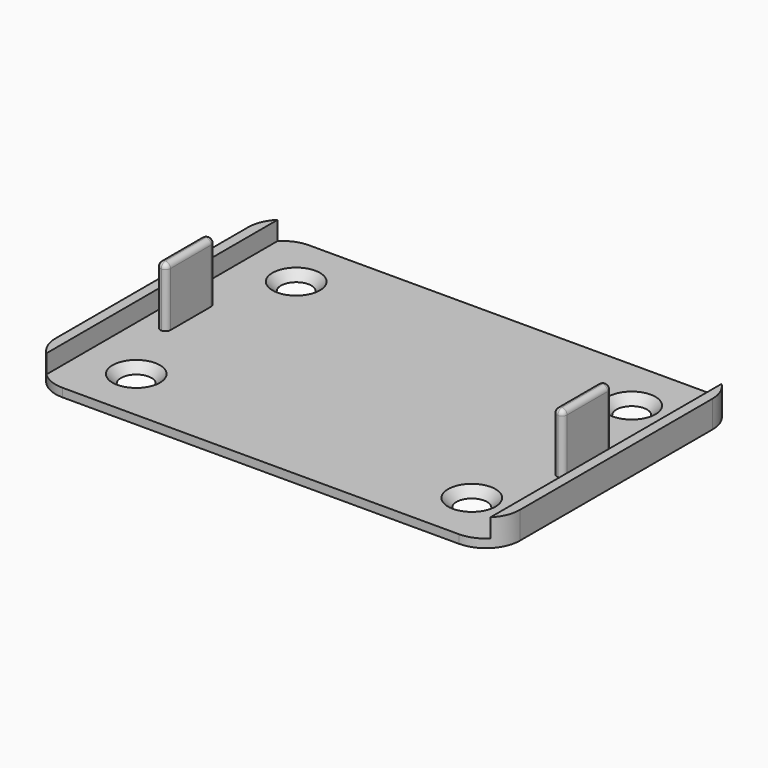
from build123d import *

# Parameters (mm, degrees)
F0_W     = 65.5
F0_H     = 45.5
F0_R     = 1.5
F0_W_2   = 1.5
F0_H_2   = 9
F1_DEPTH = 1.25
F2_DEPTH = 10
F3_DEPTH = 4
F5_R     = 0.74999
F6_R     = 0.74999
F7_R     = 5


# Not quite as in the source:
# - a fillet or chamfer that OpenCascade refuses, or shapes differently, is made with other operations: its cross-section is extruded or revolved along the edge and cut away or added
# - a fillet or chamfer is up to 0.001 mm smaller than in the source, because OpenCascade refuses the exact size


with BuildPart() as f1:
    # F0 (on Top) → F1 (new body)
    with BuildSketch(Plane.XY):
        Rectangle(F0_W, F0_H)
        with Locations((-24.75, -14.75)):
            Circle(F0_R, mode=Mode.SUBTRACT)
        with Locations((24.75, -14.75)):
            Circle(F0_R, mode=Mode.SUBTRACT)
        with Locations((-29.25, 0)):
            Rectangle(F0_W_2, F0_H_2, mode=Mode.SUBTRACT)
        with Locations((-24.75, 14.75)):
            Circle(F0_R, mode=Mode.SUBTRACT)
        with Locations((29.25, 0)):
            Rectangle(F0_W_2, F0_H_2, mode=Mode.SUBTRACT)
        with Locations((24.75, 14.75)):
            Circle(F0_R, mode=Mode.SUBTRACT)
    extrude(amount=F1_DEPTH)

    # F0 (on Top) → F2 (join)
    with BuildSketch(Plane.XY):
        with Locations((-29.25, 0)):
            Rectangle(F0_W_2, F0_H_2)
        with Locations((29.25, 0)):
            Rectangle(F0_W_2, F0_H_2)
    extrude(amount=F2_DEPTH)

    # F0 (on Top) → F3 (join)
    with BuildSketch(Plane.XY):
        with Locations((-33.5, 0)):
            Rectangle(F0_W_2, F0_H)
        with Locations((33.5, 0)):
            Rectangle(F0_W_2, F0_H)
    extrude(amount=F3_DEPTH)

    # F4: chamfer of 2 on 4 edges, made by hand

    # F4_s1 → F4_t2 (revolve, cut)
    with BuildSketch(Plane.XZ.offset(-14.75)):
        Polygon((-21.25, 1.25), (-23.25, -0.75), (-23.25, 1.25), align=None)
    revolve(axis=Axis((-24.75, 14.75, 1.25), (0, 0, 1)), mode=Mode.SUBTRACT)

    # F4_s3 → F4_t4 (revolve, cut)
    with BuildSketch(Plane.XZ.offset(14.75)):
        Polygon((-21.25, 1.25), (-23.25, -0.75), (-23.25, 1.25), align=None)
    revolve(axis=Axis((-24.75, -14.75, 1.25), (0, 0, 1)), mode=Mode.SUBTRACT)

    # F4_s5 → F4_t6 (revolve, cut)
    with BuildSketch(Plane.XZ.offset(-14.75)):
        Polygon((28.25, 1.25), (26.25, -0.75), (26.25, 1.25), align=None)
    revolve(axis=Axis((24.75, 14.75, 1.25), (0, 0, 1)), mode=Mode.SUBTRACT)

    # F4_s7 → F4_t8 (revolve, cut)
    with BuildSketch(Plane.XZ.offset(14.75)):
        Polygon((28.25, 1.25), (26.25, -0.75), (26.25, 1.25), align=None)
    revolve(axis=Axis((24.75, -14.75, 1.25), (0, 0, 1)), mode=Mode.SUBTRACT)

    # F5 (radius 0.75 in the source; OpenCascade refuses exactly that, so slightly less here)
    f5_edges = [f1.edges().sort_by_distance(p)[0] for p in [
        (-30, 4.5, 5.625),
        (30, 4.5, 5.625),
        (28.5, 4.5, 5.625),
        (-30, -4.5, 5.625),
        (-28.5, -4.5, 5.625),
        (28.5, -4.5, 5.625),
        (30, -4.5, 5.625),
        (-28.5, 4.5, 5.625),
    ]]
    fillet(f5_edges, radius=F5_R)

    # F6 (radius 0.75 in the source; OpenCascade refuses exactly that, so slightly less here)
    f6_edges = [f1.edges().sort_by_distance(p)[0] for p in [
        (-29.25, -4.5, 10),
        (-29.780333, -4.280333, 10),
        (-28.719667, -4.280333, 10),
        (-30, 0, 10),
        (-28.5, 0, 10),
        (-29.780333, 4.280333, 10),
        (-28.719667, 4.280333, 10),
        (-29.25, 4.5, 10),
        (29.25, -4.5, 10),
        (28.719667, -4.280333, 10),
        (29.780333, -4.280333, 10),
        (28.5, 0, 10),
        (30, 0, 10),
        (28.719667, 4.280333, 10),
        (29.780333, 4.280333, 10),
        (29.25, 4.5, 10),
    ]]
    fillet(f6_edges, radius=F6_R)

    # F7
    f7_edges = [f1.edges().sort_by_distance(p)[0] for p in [
        (-34.25, -22.75, 2),
        (34.25, -22.75, 2),
        (34.25, 22.75, 2),
        (-34.25, 22.75, 2),
    ]]
    fillet(f7_edges, radius=F7_R)


solid = f1.part
